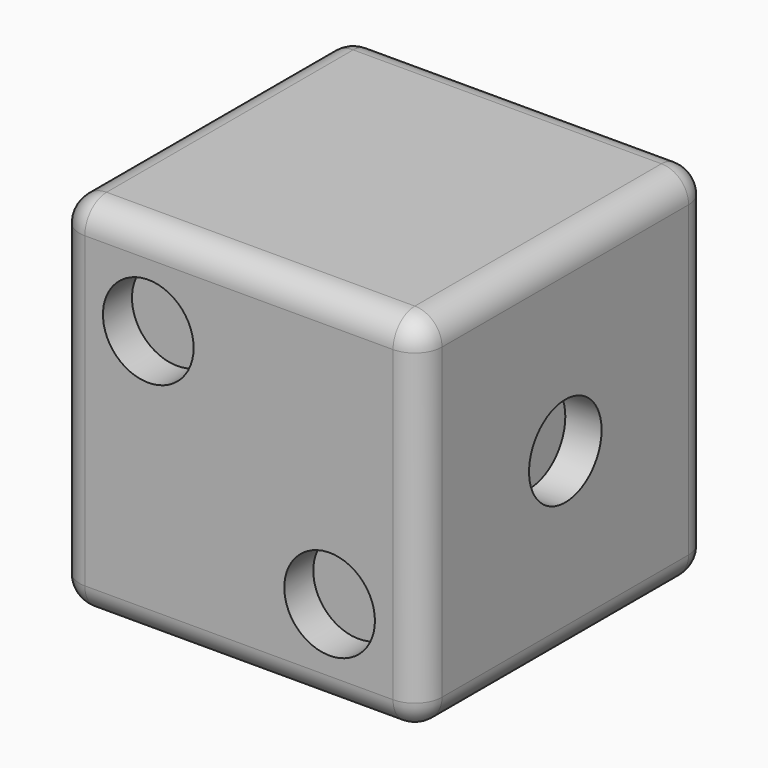
from build123d import *

# Parameters (mm, degrees)
F0_W     = 20
F0_H     = 20
F1_DEPTH = 10
F2_R     = 2.5
F3_DEPTH = 2
F4_R     = 2.5
F5_DEPTH = 2
F6_R     = 2.5
F7_DEPTH = 2
F8_R     = 1.5


# Not quite as in the source:
# - a pattern or mirror of a feature is missing from the dataset's text; its kind, count and spacing are read off the source's solid


with BuildPart() as f1:
    # F0 (on Top) → F1 (new body, symmetric)
    with BuildSketch(Plane.XY):
        Rectangle(F0_W, F0_H)
    extrude(amount=F1_DEPTH, both=True)

    # F2 (on face) → F3 (cut)
    with BuildSketch(Plane.YZ.offset(10)):
        Circle(F2_R)
    f3 = extrude(amount=-F3_DEPTH, mode=Mode.SUBTRACT)

    # F3_copies: F3 across plane
    add(f3.mirror(Plane(origin=(0, 0, 0), x_dir=(0, 0, -1), z_dir=(-1, 0, 0))), mode=Mode.SUBTRACT)

    # F4 (on face) → F5 (cut)
    with BuildSketch(Plane(origin=(0, 10, 0), x_dir=(-1, 0, 0), z_dir=(0, 1, 0))):
        with Locations((5, -5)):
            Circle(F4_R)
        with Locations((-5, 5)):
            Circle(F4_R)
    extrude(amount=-F5_DEPTH, mode=Mode.SUBTRACT)

    # F6 (on face) → F7 (cut)
    with BuildSketch(Plane.XZ.offset(10)):
        with Locations((-5, 5)):
            Circle(F6_R)
        with Locations((5, -5)):
            Circle(F6_R)
    extrude(amount=-F7_DEPTH, mode=Mode.SUBTRACT)

    # F8
    f8_edges = [f1.edges().sort_by_distance(p)[0] for p in [
        (10, 0, 10),
        (0, 10, 10),
        (10, 10, 0),
        (10, -10, 0),
        (10, 0, -10),
        (0, -10, -10),
        (-10, 0, -10),
        (0, 10, -10),
        (-10, 10, 0),
        (-10, -10, 0),
        (0, -10, 10),
        (-10, 0, 10),
    ]]
    fillet(f8_edges, radius=F8_R)


solid = f1.part
